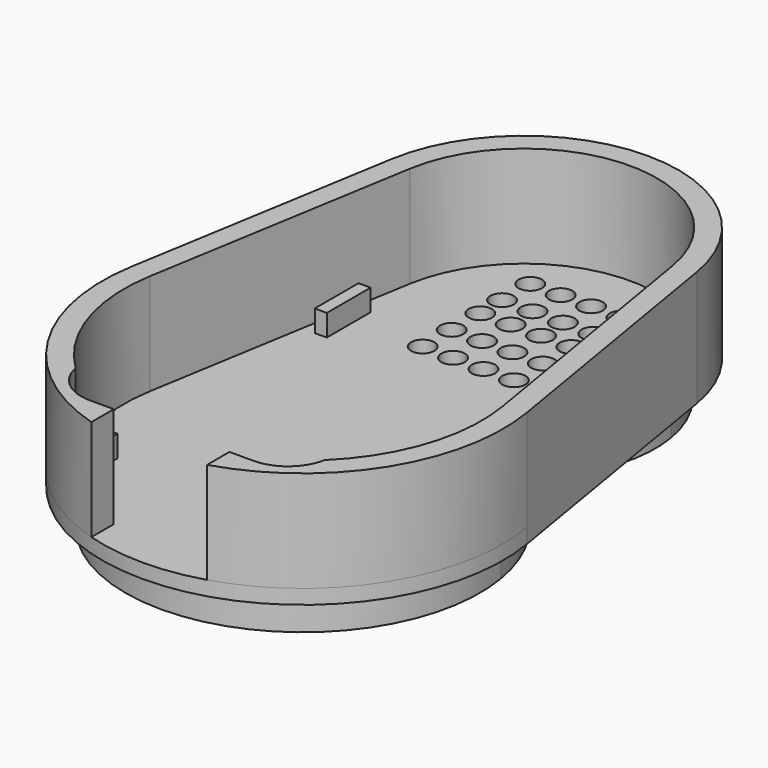
from build123d import *

# Parameters (mm, degrees)
F1_DEPTH = 1
F2_DEPTH = 3.5
F4_DEPTH = 7
F3_W     = 0.8317038625
F3_H     = 3.7825570011
F3_W_2   = 0.7836289912
F3_W_3   = 0.6960576609
F3_H_2   = 2.5395583361
F3_W_4   = 0.6565612018
F5_DEPTH = 1.5
F3_R     = 0.8088750424
F6_DEPTH = 5


with BuildPart() as f1:
    # F0 (on Top) → F1 (new body)
    with BuildSketch(Plane.XY):
        with BuildLine():
            ThreePointArc((10.5534817095, 15.4336250836), (0, 24.3689653978), (-10.5534817095, 15.4336250836))
            Line((-10.5534817095, 15.4336250836), (-13.6603478203, -3.1468722986))
            ThreePointArc((-13.6603478203, -3.1468722986), (0, -19.2810346022), (13.6603478203, -3.1468722986))
            Line((13.6603478203, -3.1468722986), (10.5534817095, 15.4336250836))
        make_face()
        with BuildLine():
            ThreePointArc((-7.9318843768, 3.9042591925), (-7.9136479922, 3.9365495997), (-7.8956354366, 3.9689653978))
            ThreePointArc((-7.8956354366, 3.9689653978), (-7.2435768772, 6.1726329025), (-7.5742542147, 8.4468323957))
            ThreePointArc((-7.5742542147, 8.4468323957), (-7.7343170695, 8.8265985648), (-7.9230829656, 9.1929452547))
            ThreePointArc((-7.9230829656, 9.1929452547), (-8.9621513279, 12.0910415797), (-8.9753909866, 15.1697507381))
            ThreePointArc((-8.9753909866, 15.1697507381), (0, 22.7689653978), (8.9753909866, 15.1697507381))
            ThreePointArc((8.9753909866, 15.1697507381), (8.9621513279, 12.0910415797), (7.9230829656, 9.1929452547))
            ThreePointArc((7.9230829656, 9.1929452547), (7.7343170695, 8.8265985648), (7.5742542147, 8.4468323957))
            ThreePointArc((7.5742542147, 8.4468323957), (7.2435768772, 6.1726329025), (7.8956354366, 3.9689653978))
            ThreePointArc((7.8956354366, 3.9689653978), (7.9136479922, 3.9365495997), (7.9318843768, 3.9042591925))
            ThreePointArc((7.9318843768, 3.9042591925), (10.6545198078, 0.6141045745), (12.0822570973, -3.4107466441))
            ThreePointArc((12.0822570973, -3.4107466441), (0, -17.6810346022), (-12.0822570973, -3.4107466441))
            ThreePointArc((-12.0822570973, -3.4107466441), (-10.6545198078, 0.6141045745), (-7.9318843768, 3.9042591925))
        make_face(mode=Mode.SUBTRACT)
        with BuildLine():
            Line((7.8956354366, 3.9689653978), (-7.8956354366, 3.9689653978))
            ThreePointArc((-7.8956354366, 3.9689653978), (-7.9136479922, 3.9365495997), (-7.9318843768, 3.9042591925))
            ThreePointArc((-7.9318843768, 3.9042591925), (-10.6545198078, 0.6141045745), (-12.0822570973, -3.4107466441))
            ThreePointArc((-12.0822570973, -3.4107466441), (0, -17.6810346022), (12.0822570973, -3.4107466441))
            ThreePointArc((12.0822570973, -3.4107466441), (10.6545198078, 0.6141045745), (7.9318843768, 3.9042591925))
            ThreePointArc((7.9318843768, 3.9042591925), (7.9136479922, 3.9365495997), (7.8956354366, 3.9689653978))
        make_face()
        with BuildLine():
            ThreePointArc((-7.9230829656, 9.1929452547), (-7.7343170695, 8.8265985648), (-7.5742542147, 8.4468323957))
            ThreePointArc((-7.5742542147, 8.4468323957), (0, 4.4689653978), (7.5742542147, 8.4468323957))
            ThreePointArc((7.5742542147, 8.4468323957), (7.7343170695, 8.8265985648), (7.9230829656, 9.1929452547))
            ThreePointArc((7.9230829656, 9.1929452547), (8.9621513279, 12.0910415797), (8.9753909866, 15.1697507381))
            ThreePointArc((8.9753909866, 15.1697507381), (0, 22.7689653978), (-8.9753909866, 15.1697507381))
            ThreePointArc((-8.9753909866, 15.1697507381), (-8.9621513279, 12.0910415797), (-7.9230829656, 9.1929452547))
        make_face()
        with BuildLine():
            ThreePointArc((-7.5742542147, 8.4468323957), (-7.2435768772, 6.1726329025), (-7.8956354366, 3.9689653978))
            Line((-7.8956354366, 3.9689653978), (7.8956354366, 3.9689653978))
            ThreePointArc((7.8956354366, 3.9689653978), (7.2435768772, 6.1726329025), (7.5742542147, 8.4468323957))
            ThreePointArc((7.5742542147, 8.4468323957), (0, 4.4689653978), (-7.5742542147, 8.4468323957))
        make_face()
    extrude(amount=-F1_DEPTH)

    # F0 (on Top) → F2 (join)
    with BuildSketch(Plane.XY):
        with BuildLine():
            ThreePointArc((-7.5742542147, 8.4468323957), (-7.2435768772, 6.1726329025), (-7.8956354366, 3.9689653978))
            Line((-7.8956354366, 3.9689653978), (7.8956354366, 3.9689653978))
            ThreePointArc((7.8956354366, 3.9689653978), (7.2435768772, 6.1726329025), (7.5742542147, 8.4468323957))
            ThreePointArc((7.5742542147, 8.4468323957), (0, 4.4689653978), (-7.5742542147, 8.4468323957))
        make_face()
        with BuildLine():
            Line((7.8956354366, 3.9689653978), (-7.8956354366, 3.9689653978))
            ThreePointArc((-7.8956354366, 3.9689653978), (-7.9136479922, 3.9365495997), (-7.9318843768, 3.9042591925))
            ThreePointArc((-7.9318843768, 3.9042591925), (-10.6545198078, 0.6141045745), (-12.0822570973, -3.4107466441))
            ThreePointArc((-12.0822570973, -3.4107466441), (0, -17.6810346022), (12.0822570973, -3.4107466441))
            ThreePointArc((12.0822570973, -3.4107466441), (10.6545198078, 0.6141045745), (7.9318843768, 3.9042591925))
            ThreePointArc((7.9318843768, 3.9042591925), (7.9136479922, 3.9365495997), (7.8956354366, 3.9689653978))
        make_face()
        with BuildLine():
            ThreePointArc((-7.9230829656, 9.1929452547), (-7.7343170695, 8.8265985648), (-7.5742542147, 8.4468323957))
            ThreePointArc((-7.5742542147, 8.4468323957), (0, 4.4689653978), (7.5742542147, 8.4468323957))
            ThreePointArc((7.5742542147, 8.4468323957), (7.7343170695, 8.8265985648), (7.9230829656, 9.1929452547))
            ThreePointArc((7.9230829656, 9.1929452547), (8.9621513279, 12.0910415797), (8.9753909866, 15.1697507381))
            ThreePointArc((8.9753909866, 15.1697507381), (0, 22.7689653978), (-8.9753909866, 15.1697507381))
            ThreePointArc((-8.9753909866, 15.1697507381), (-8.9621513279, 12.0910415797), (-7.9230829656, 9.1929452547))
        make_face()
    extrude(amount=-F2_DEPTH)

    # F3 (on face) → F4 (join)
    with BuildSketch(Plane.XY):
        with BuildLine():
            Line((-4, -16.7553447357), (-5.65, -16.7553447357))
            ThreePointArc((-5.65, -16.7553447357), (-7.5717587133, -16.0590034448), (-8.6013841311, -14.2932403677))
            ThreePointArc((-8.6013841311, -14.2932403677), (-11.7334001707, -9.284581077), (-12.1808877675, -3.3942544975))
            Line((-12.1808877675, -3.3942544975), (-9.0740216568, 15.1862428847))
            ThreePointArc((-9.0740216568, 15.1862428847), (0, 22.8689653978), (9.0740216568, 15.1862428847))
            Line((9.0740216568, 15.1862428847), (12.1808877675, -3.3942544975))
            ThreePointArc((12.1808877675, -3.3942544975), (11.7334001707, -9.284581077), (8.6013841311, -14.2932403677))
            ThreePointArc((8.6013841311, -14.2932403677), (7.5717587133, -16.0590034448), (5.65, -16.7553447357))
            Line((5.65, -16.7553447357), (4, -16.7553447357))
            Line((4, -16.7553447357), (4, -17.9553447357))
            Line((4, -17.9553447357), (4, -18.6908422931))
            ThreePointArc((4, -18.6908422931), (11.7633210481, -12.7417649295), (13.6603478203, -3.1468722986))
            Line((13.6603478203, -3.1468722986), (10.5534817095, 15.4336250836))
            ThreePointArc((10.5534817095, 15.4336250836), (0, 24.3689653978), (-10.5534817095, 15.4336250836))
            Line((-10.5534817095, 15.4336250836), (-13.6603478203, -3.1468722986))
            ThreePointArc((-13.6603478203, -3.1468722986), (-11.7633210481, -12.7417649295), (-4, -18.6908422931))
            Line((-4, -18.6908422931), (-4, -17.9553447357))
            Line((-4, -17.9553447357), (-4, -16.7553447357))
        make_face()
    extrude(amount=F4_DEPTH)

    # F3 (on face) → F5 (join)
    with BuildSketch(Plane.XY):
        with Locations((-9.0658519313, 9.3533767637)):
            Rectangle(F3_W, F3_H)
        with Locations((9.0418144956, 9.3533767637)):
            Rectangle(F3_W_2, F3_H)
        with Locations((8.9980288304, -11.8910893798)):
            Rectangle(F3_W_3, F3_H_2)
        with Locations((-8.9782806009, -11.8910893798)):
            Rectangle(F3_W_4, F3_H_2)
    extrude(amount=F5_DEPTH)

    # F3 (on face) → F6 (cut)
    with BuildSketch(Plane.XY):
        with Locations((-3.9931656793, 19.2196834832)):
            Circle(F3_R)
        with Locations((-1.8931656793, 19.2196834832)):
            Circle(F3_R)
        with Locations((0.2068343207, 19.2196834832)):
            Circle(F3_R)
        with Locations((2.3068343207, 19.2196834832)):
            Circle(F3_R)
        with Locations((4.4068343207, 19.2196834832)):
            Circle(F3_R)
        with Locations((4.4068343207, 16.7862419039)):
            Circle(F3_R)
        with Locations((2.3068343207, 16.7862419039)):
            Circle(F3_R)
        with Locations((0.2068343207, 16.7862419039)):
            Circle(F3_R)
        with Locations((-1.8931656793, 16.7862419039)):
            Circle(F3_R)
        with Locations((-3.9931656793, 16.7862419039)):
            Circle(F3_R)
        with Locations((-3.9502955042, 14.8469135165)):
            Circle(F3_R)
        with Locations((-1.8502955042, 14.8469135165)):
            Circle(F3_R)
        with Locations((0.2497044958, 14.8469135165)):
            Circle(F3_R)
        with Locations((2.3497044958, 14.8469135165)):
            Circle(F3_R)
        with Locations((4.4497044958, 14.8469135165)):
            Circle(F3_R)
        with Locations((-3.9502955042, 12.3752485961)):
            Circle(F3_R)
        with Locations((-1.8502955042, 12.3752485961)):
            Circle(F3_R)
        with Locations((0.2497044958, 12.3752485961)):
            Circle(F3_R)
        with Locations((2.3497044958, 12.3752485961)):
            Circle(F3_R)
        with Locations((4.4497044958, 12.3752485961)):
            Circle(F3_R)
        with Locations((-3.9502955042, 9.8736844957)):
            Circle(F3_R)
        with Locations((-1.8502955042, 9.8736844957)):
            Circle(F3_R)
        with Locations((0.2497044958, 9.8736844957)):
            Circle(F3_R)
        with Locations((2.3497044958, 9.8736844957)):
            Circle(F3_R)
        with Locations((4.4497044958, 9.8736844957)):
            Circle(F3_R)
    extrude(amount=-F6_DEPTH, mode=Mode.SUBTRACT)


solid = f1.part
